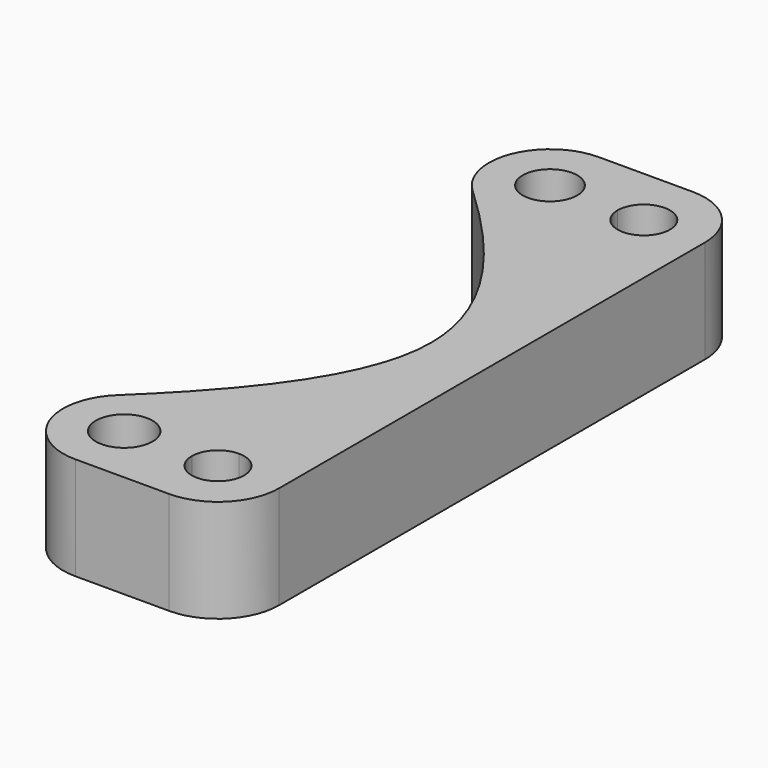
from build123d import *

# Parameters (mm, degrees)
F0_R     = 6.25
F0_R_2   = 6.5
F1_DEPTH = 23.6


# Not quite as in the source:
# - a feature names something its author has since deleted; it is built from what else it names


with BuildPart() as f1:
    # F0 (on Top) → F1 (new body)
    with BuildSketch(Plane.XY):
        with BuildLine():
            ThreePointArc((-40.3365694268, 61), (-34.3365694268, 67), (-28.3365694268, 61))
            ThreePointArc((-28.3365694268, 61), (-30.0939287397, 56.7573593129), (-34.3365694268, 55))
            Line((-34.3365694268, 55), (-34.3365694268, 47))
            ThreePointArc((-34.3365694268, 47), (-24.4370744902, 51.1005050634), (-20.3365694268, 61))
            ThreePointArc((-20.3365694268, 61), (-24.4370744902, 70.8994949366), (-34.3365694268, 75))
            ThreePointArc((-34.3365694268, 75), (-40.2711402705, 73.6799396253), (-45.0865694268, 69.9686955573))
            ThreePointArc((-45.0865694268, 69.9686955573), (-42.6741228457, 65.7696960071), (-41.8365694268, 61))
            Line((-41.8365694268, 61), (-40.3365694268, 61))
        make_face()
        with BuildLine():
            ThreePointArc((-20.3365694268, 61), (-24.4370744902, 51.1005050634), (-34.3365694268, 47))
            Line((-34.3365694268, 47), (-34.3365694268, 0.2172092025))
            add(Edge.make_bspline(
                [(-34.3365694268, 0.2172092025), (-34.3363249407, 0.1448037453), (-34.3363246716, 0.0724006335), (-34.3365694268, 0)],
                knots=[0.4978036396, 0.4978036396, 0.4978036396, 0.4978036396, 0.4996491669, 0.4996491669, 0.4996491669, 0.4996491669], degree=3))
            Line((-34.3365694268, 0), (-34.3365694268, -47))
            ThreePointArc((-34.3365694268, -47), (-24.4370744902, -51.1005050634), (-20.3365694268, -61))
            Line((-20.3365694268, -61), (-20.3365694268, 61))
        make_face()
        with BuildLine():
            Line((-34.3365694268, 0.2172092025), (-34.3365694268, 47))
            ThreePointArc((-34.3365694268, 47), (-40.2711402705, 48.3200603747), (-45.0865694268, 52.0313044427))
            ThreePointArc((-45.0865694268, 52.0313044427), (-54.9532680212, 47.0278928351), (-65.3715156462, 50.7489122239))
            add(Edge.make_bspline(
                [(-65.3715156462, 50.7489122239), (-48.4197455884, 34.9813943951), (-34.3950357775, 17.5322350251), (-34.3365694268, 0.2172092025)],
                knots=[0.0564646149, 0.0564646149, 0.0564646149, 0.0564646149, 0.4978036396, 0.4978036396, 0.4978036396, 0.4978036396], degree=3))
        make_face()
        with BuildLine():
            ThreePointArc((-45.0865694268, 52.0313044427), (-47.4990160079, 56.2303039929), (-48.3365694268, 61))
            ThreePointArc((-48.3365694268, 61), (-47.4990160079, 65.7696960071), (-45.0865694268, 69.9686955573))
            ThreePointArc((-45.0865694268, 69.9686955573), (-49.9019985831, 73.6799396253), (-55.8365694268, 75))
            ThreePointArc((-55.8365694268, 75), (-68.8656758594, 66.1227322365), (-65.3715156462, 50.7489122239))
            ThreePointArc((-65.3715156462, 50.7489122239), (-54.9532680212, 47.0278928351), (-45.0865694268, 52.0313044427))
        make_face()
        with Locations((-55.8365694268, 61)):
            Circle(F0_R, mode=Mode.SUBTRACT)
        with BuildLine():
            ThreePointArc((-55.8365694268, 75), (-49.9019985831, 73.6799396253), (-45.0865694268, 69.9686955573))
            ThreePointArc((-45.0865694268, 69.9686955573), (-40.2711402705, 73.6799396253), (-34.3365694268, 75))
            Line((-34.3365694268, 75), (-55.8365694268, 75))
        make_face()
        with BuildLine():
            add(Edge.make_bspline(
                [(-34.3365694268, 0.2172092025), (-34.3363249407, 0.1448037453), (-34.3363246716, 0.0724006335), (-34.3365694268, 0)],
                knots=[0.4978036396, 0.4978036396, 0.4978036396, 0.4978036396, 0.4996491669, 0.4996491669, 0.4996491669, 0.4996491669], degree=3))
            Line((-34.3365694268, 0.2172092025), (-34.3365694268, 0))
        make_face()
        with BuildLine():
            Line((-34.3365694268, -47), (-34.3365694268, 0))
            add(Edge.make_bspline(
                [(-34.3365694268, 0), (-34.3955070338, -17.4342401848), (-48.662358916, -34.7247764323), (-65.5260679692, -50.8948716982)],
                knots=[0.4996491669, 0.4996491669, 0.4996491669, 0.4996491669, 0.9440564283, 0.9440564283, 0.9440564283, 0.9440564283], degree=3))
            ThreePointArc((-65.5260679692, -50.8948716982), (-55.0593721024, -47.0215893493), (-45.0865694268, -52.0313044427))
            ThreePointArc((-45.0865694268, -52.0313044427), (-40.2711402705, -48.3200603747), (-34.3365694268, -47))
        make_face()
        with BuildLine():
            ThreePointArc((-34.3365694268, -75), (-24.4370744902, -70.8994949366), (-20.3365694268, -61))
            ThreePointArc((-20.3365694268, -61), (-24.4370744902, -51.1005050634), (-34.3365694268, -47))
            Line((-34.3365694268, -47), (-34.3365694268, -55))
            ThreePointArc((-34.3365694268, -55), (-30.0939287397, -56.7573593129), (-28.3365694268, -61))
            ThreePointArc((-28.3365694268, -61), (-34.3365694268, -67), (-40.3365694268, -61))
            Line((-40.3365694268, -61), (-41.8365694268, -61))
            ThreePointArc((-41.8365694268, -61), (-42.6741228457, -65.7696960071), (-45.0865694268, -69.9686955573))
            ThreePointArc((-45.0865694268, -69.9686955573), (-40.2711402705, -73.6799396253), (-34.3365694268, -75))
        make_face()
        with BuildLine():
            ThreePointArc((-45.0865694268, -52.0313044427), (-55.0593721024, -47.0215893493), (-65.5260679692, -50.8948716982))
            ThreePointArc((-65.5260679692, -50.8948716982), (-68.8264076903, -66.2215037956), (-55.8365694268, -75))
            ThreePointArc((-55.8365694268, -75), (-49.9019985831, -73.6799396253), (-45.0865694268, -69.9686955573))
            ThreePointArc((-45.0865694268, -69.9686955573), (-47.4990160079, -65.7696960071), (-48.3365694268, -61))
            ThreePointArc((-48.3365694268, -61), (-47.4990160079, -56.2303039929), (-45.0865694268, -52.0313044427))
        make_face()
        with Locations((-55.8365694268, -61)):
            Circle(F0_R_2, mode=Mode.SUBTRACT)
        with BuildLine():
            Line((-55.8365694268, -75), (-34.3365694268, -75))
            ThreePointArc((-34.3365694268, -75), (-40.2711402705, -73.6799396253), (-45.0865694268, -69.9686955573))
            ThreePointArc((-45.0865694268, -69.9686955573), (-49.9019985831, -73.6799396253), (-55.8365694268, -75))
        make_face()
        with BuildLine():
            ThreePointArc((-34.3365694268, 55), (-38.5792101139, 56.7573593129), (-40.3365694268, 61))
            Line((-40.3365694268, 61), (-41.8365694268, 61))
            ThreePointArc((-41.8365694268, 61), (-42.6741228457, 56.2303039929), (-45.0865694268, 52.0313044427))
            ThreePointArc((-45.0865694268, 52.0313044427), (-40.2711402705, 48.3200603747), (-34.3365694268, 47))
            Line((-34.3365694268, 47), (-34.3365694268, 55))
        make_face()
        with BuildLine():
            Line((-48.3365694268, 61), (-41.8365694268, 61))
            ThreePointArc((-41.8365694268, 61), (-42.6741228457, 65.7696960071), (-45.0865694268, 69.9686955573))
            ThreePointArc((-45.0865694268, 69.9686955573), (-47.4990160079, 65.7696960071), (-48.3365694268, 61))
        make_face()
        with BuildLine():
            ThreePointArc((-45.0865694268, 52.0313044427), (-42.6741228457, 56.2303039929), (-41.8365694268, 61))
            Line((-41.8365694268, 61), (-48.3365694268, 61))
            ThreePointArc((-48.3365694268, 61), (-47.4990160079, 56.2303039929), (-45.0865694268, 52.0313044427))
        make_face()
        with BuildLine():
            Line((-34.3365694268, -55), (-34.3365694268, -47))
            ThreePointArc((-34.3365694268, -47), (-40.2711402705, -48.3200603747), (-45.0865694268, -52.0313044427))
            ThreePointArc((-45.0865694268, -52.0313044427), (-42.6741228457, -56.2303039929), (-41.8365694268, -61))
            Line((-41.8365694268, -61), (-40.3365694268, -61))
            ThreePointArc((-40.3365694268, -61), (-38.5792101139, -56.7573593129), (-34.3365694268, -55))
        make_face()
        with BuildLine():
            ThreePointArc((-41.8365694268, -61), (-42.6741228457, -56.2303039929), (-45.0865694268, -52.0313044427))
            ThreePointArc((-45.0865694268, -52.0313044427), (-47.4990160079, -56.2303039929), (-48.3365694268, -61))
            Line((-48.3365694268, -61), (-41.8365694268, -61))
        make_face()
        with BuildLine():
            ThreePointArc((-48.3365694268, -61), (-47.4990160079, -65.7696960071), (-45.0865694268, -69.9686955573))
            ThreePointArc((-45.0865694268, -69.9686955573), (-42.6741228457, -65.7696960071), (-41.8365694268, -61))
            Line((-41.8365694268, -61), (-48.3365694268, -61))
        make_face()
    extrude(amount=F1_DEPTH)


solid = f1.part
